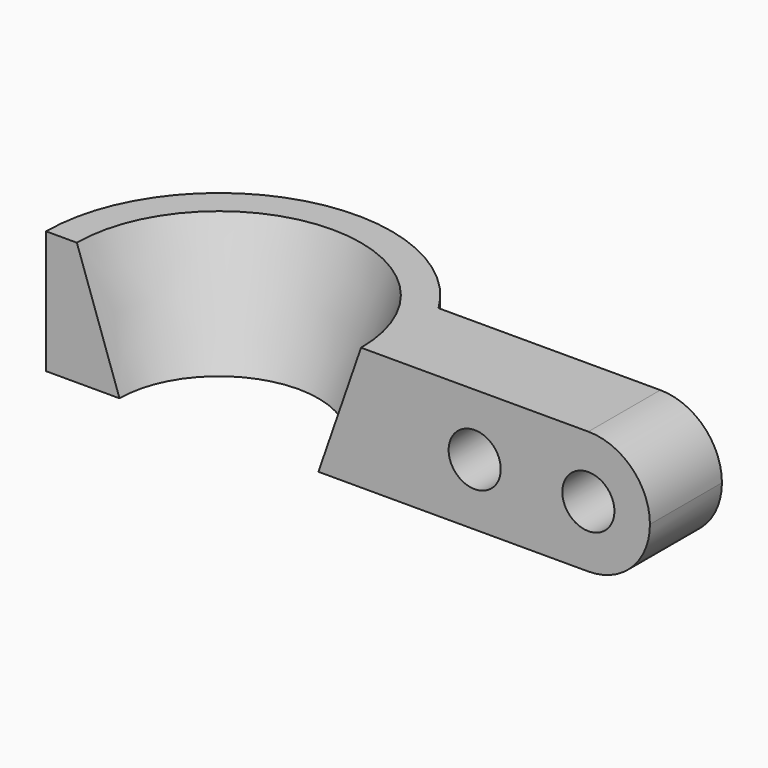
from build123d import *

# Parameters (mm, degrees)
F1_DEPTH = 52
F4_R     = 11
F5_DEPTH = 57
F6_R     = 25.99999


# Not quite as in the source:
# - a fillet or chamfer is up to 0.001 mm smaller than in the source, because OpenCascade refuses the exact size


with BuildPart() as f1:
    # F0 (on Top) → F1 (new body)
    with BuildSketch(Plane.XY):
        with BuildLine():
            Line((182, 38), (62.329768169, 38))
            ThreePointArc((62.329768169, 38), (-19.7348286497, 70.2818364741), (-73, 0))
            Line((-73, 0), (-42, 0))
            ThreePointArc((-42, 0), (0, 42), (42, 0))
            Line((42, 0), (182, 0))
            Line((182, 0), (182, 38))
        make_face()
    extrude(amount=F1_DEPTH)

    # F2 (on Front) → F3 (revolve, cut)
    with BuildSketch(Plane.XZ):
        Polygon((-42, 0), (0, 0), (0, 52), (-60, 52), align=None)
    revolve(axis=Axis((0, 0, 26), (0, 0, 1)), mode=Mode.SUBTRACT)

    # F4 (on face) → F5 (cut)
    with BuildSketch(Plane.XZ):
        with Locations((108, 26)):
            Circle(F4_R)
        with Locations((156, 26)):
            Circle(F4_R)
    extrude(amount=-F5_DEPTH, mode=Mode.SUBTRACT)

    # F6 (radius 26 in the source; OpenCascade refuses exactly that, so slightly less here)
    f6_edges = [f1.edges().sort_by_distance(p)[0] for p in [
        (182, 19, 52),
        (182, 19, 0),
    ]]
    fillet(f6_edges, radius=F6_R)


solid = f1.part
